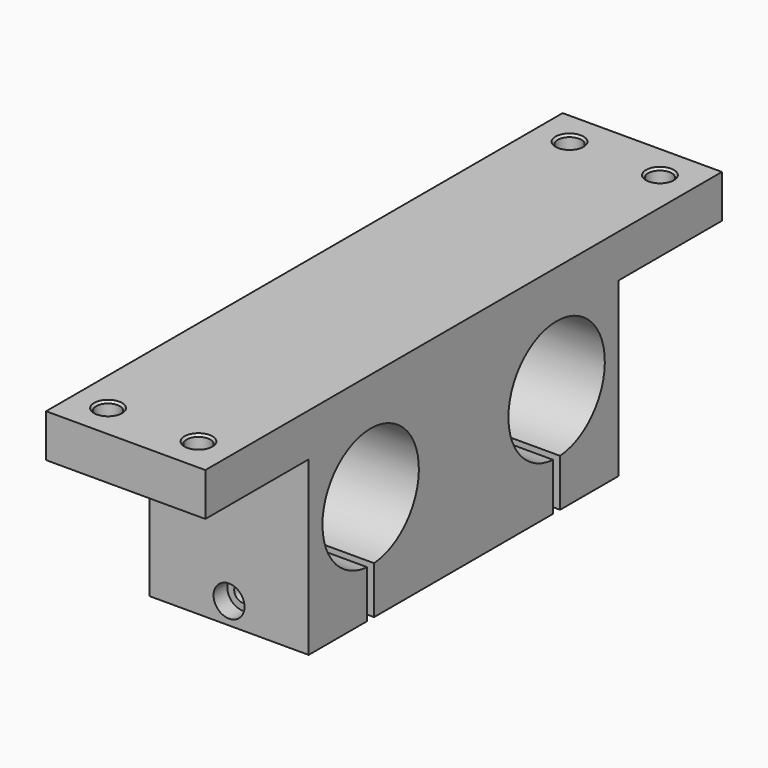
from build123d import *

# Parameters (mm, degrees)
F1_DEPTH  = 37
F2_R      = 2
F3_DEPTH  = 30
F4_R      = 3.6
F5_DEPTH  = 4
F6_R      = 2
F7_DEPTH  = 30
F8_R      = 3.6
F9_DEPTH  = 4
F10_R     = 2.75
F11_DEPTH = 50.001
F12_SIZE  = 0.5


with BuildPart() as f1:
    # F0 (on Right) → F1 (new body)
    with BuildSketch(Plane.YZ):
        with BuildLine():
            Line((-45, 0), (-45, -40))
            Line((-45, -40), (-28, -40))
            Line((-28, -40), (-28, -28.9642400438))
            ThreePointArc((-28, -28.9642400438), (-27, -1), (-26, -28.9642400438))
            Line((-26, -28.9642400438), (-26, -40))
            Line((-26, -40), (26, -40))
            Line((26, -40), (26, -28.9642400438))
            ThreePointArc((26, -28.9642400438), (27, -1), (28, -28.9642400438))
            Line((28, -28.9642400438), (28, -40))
            Line((28, -40), (45, -40))
            Line((45, -40), (45, 0))
            Line((45, 0), (75, 0))
            Line((75, 0), (75, 10))
            Line((75, 10), (-75, 10))
            Line((-75, 10), (-75, 0))
            Line((-75, 0), (-45, 0))
        make_face()
    extrude(amount=F1_DEPTH)

    # F2 (on face) → F3 (cut)
    with BuildSketch(Plane.XZ.offset(45)):
        with Locations((18.5, -35)):
            Circle(F2_R)
    extrude(amount=-F3_DEPTH, mode=Mode.SUBTRACT)

    # F4 (on face) → F5 (cut)
    with BuildSketch(Plane.XZ.offset(45)):
        with Locations((18.5, -35)):
            Circle(F4_R)
    extrude(amount=-F5_DEPTH, mode=Mode.SUBTRACT)

    # F6 (on face) → F7 (cut)
    with BuildSketch(Plane(origin=(0, 45, 0), x_dir=(-1, 0, 0), z_dir=(0, 1, 0))):
        with Locations((-18.5, -35)):
            Circle(F6_R)
    extrude(amount=-F7_DEPTH, mode=Mode.SUBTRACT)

    # F8 (on face) → F9 (cut)
    with BuildSketch(Plane(origin=(0, 45, 0), x_dir=(-1, 0, 0), z_dir=(0, 1, 0))):
        with Locations((-18.5, -35)):
            Circle(F8_R)
    extrude(amount=-F9_DEPTH, mode=Mode.SUBTRACT)

    # F10 (on face) → F11 (cut, through all)
    with BuildSketch(Plane.XY.offset(10)):
        with Locations((29, 67)):
            Circle(F10_R)
        with Locations((8, 67)):
            Circle(F10_R)
        with Locations((8, -67)):
            Circle(F10_R)
        with Locations((29, -67)):
            Circle(F10_R)
    extrude(amount=-F11_DEPTH, mode=Mode.SUBTRACT)

    # F12
    f12_edges = [f1.edges().sort_by_distance(p)[0] for p in [
        (5.25, 67, 10),
        (10.75, 67, 5),
        (5.25, 67, 0),
        (26.25, 67, 10),
        (31.75, 67, 5),
        (26.25, 67, 0),
        (5.25, -67, 10),
        (10.75, -67, 5),
        (5.25, -67, 0),
        (26.25, -67, 10),
        (31.75, -67, 5),
        (26.25, -67, 0),
    ]]
    chamfer(f12_edges, length=F12_SIZE)


solid = f1.part
